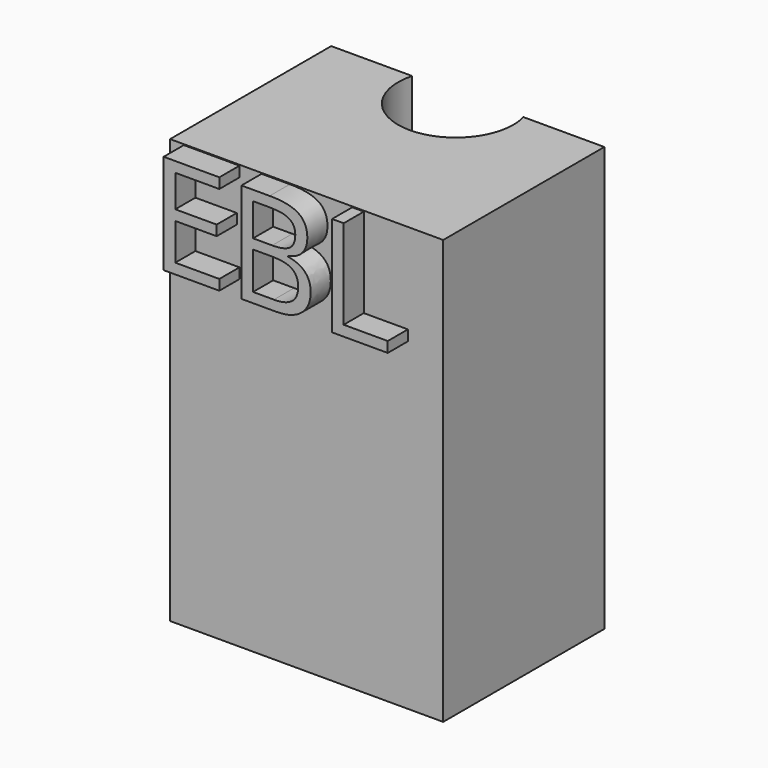
from build123d import *

# Parameters (mm, degrees)
F1_DEPTH     = 42.13
F2_TEXT_SIZE = 13.8888888889
F3_DEPTH     = 2.5


# Not quite as in the source:
# - Text() gives the source's letters only with a copy of the font that has no kerning and outlines rounded to 1/6400 em; it was checked with that copy


with BuildPart() as f1:
    # F0 (on Top) → F1 (new body)
    with BuildSketch(Plane.XY):
        with BuildLine():
            Line((-13.56, -10), (13.56, -10))
            Line((13.56, -10), (13.56, 10))
            Line((13.56, 10), (5.525, 10))
            ThreePointArc((5.525, 10), (5.6747797314, 9.2566372975), (5.725, 8.5))
            ThreePointArc((5.725, 8.5), (-0.7566372975, 2.8252202686), (-5.525, 10))
            Line((-5.525, 10), (-13.56, 10))
            Line((-13.56, 10), (-13.56, -10))
        make_face()
    extrude(amount=F1_DEPTH)

    # F2 (on face) → F3 (join)
    with BuildSketch(Plane.XZ.offset(10)):
        with Locations((-13.56, 32.13)):
            Text('EBL', F2_TEXT_SIZE, font='Open Sans', text_align=(TextAlign.LEFT, TextAlign.BOTTOM))
    extrude(amount=F3_DEPTH)


solid = f1.part
